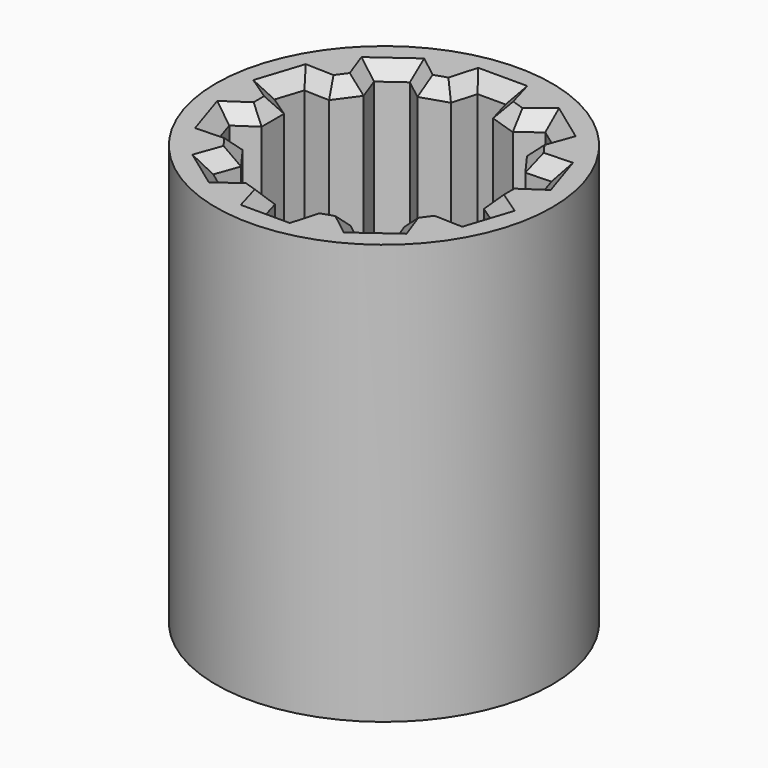
from build123d import *

# Parameters (mm, degrees)
F0_R     = 6
F1_DEPTH = 15
F2_SIZE  = 0.5


# Not quite as in the source:
# - a feature names something its author has since deleted; it is built from what else it names


with BuildPart() as f1:
    # F0 (on Top) → F1 (new body)
    with BuildSketch(Plane.XY):
        Circle(F0_R)
        Polygon((0.5, 4.8), (0.7508449189, 3.9288970345), (1.7019014352, 3.6198800401), (2.4168607138, 4.1771741991), (3.2258777082, 3.5893889469), (2.9167940342, 2.7372089), (3.5045792865, 1.9281919056), (4.410562781, 1.9588098311), (4.7195797754, 1.0077533149), (3.9686269666, 0.5), (3.9686269666, -0.5), (4.7195797754, -1.0077533149), (4.410562781, -1.9588098311), (3.5045792865, -1.9281919056), (2.9167940342, -2.7372089), (3.2258777082, -3.5893889469), (2.4168607138, -4.1771741991), (1.7019014352, -3.6198800401), (0.7508449189, -3.9288970345), (0.5, -4.8), (-0.5, -4.8), (-0.7508449189, -3.9288970345), (-1.7019014352, -3.6198800401), (-2.4168607138, -4.1771741991), (-3.2258777082, -3.5893889469), (-2.9167940342, -2.7372089), (-3.5045792865, -1.9281919056), (-4.410562781, -1.9588098311), (-4.7195797754, -1.0077533149), (-3.9686269666, -0.5), (-3.9686269666, 0.5), (-4.7195797754, 1.0077533149), (-4.410562781, 1.9588098311), (-3.5045792865, 1.9281919056), (-2.9167940342, 2.7372089), (-3.2258777082, 3.5893889469), (-2.4168607138, 4.1771741991), (-1.7019014352, 3.6198800401), (-0.7508449189, 3.9288970345), (-0.5, 4.8), align=None, mode=Mode.SUBTRACT)
    extrude(amount=F1_DEPTH)

    # F2
    f2_edges = [f1.edges().sort_by_distance(p)[0] for p in [
        (-3.071336, -3.163299, 15),
        (-1.226373, -3.774389, 15),
        (-4.565071, -1.483282, 15),
        (-4.565071, 1.483282, 15),
        (-2.821369, -3.883282, 15),
        (-4.344103, 0.753877, 15),
        (2.821369, 3.883282, 15),
        (-0.625422, -4.364449, 15),
        (-3.210687, -2.3327, 15),
        (-3.071336, 3.163299, 15),
        (1.226373, -3.774389, 15),
        (-4.344103, -0.753877, 15),
        (2.059381, 3.898527, 15),
        (3.071336, -3.163299, 15),
        (4.565071, 1.483282, 15),
        (3.957571, 1.943501, 15),
        (3.968627, 0, 15),
        (3.071336, 3.163299, 15),
        (4.344103, 0.753877, 15),
        (2.821369, -3.883282, 15),
        (3.210687, 2.3327, 15),
        (0.625422, 4.364449, 15),
        (-2.059381, 3.898527, 15),
        (0, 4.8, 15),
        (3.957571, -1.943501, 15),
        (2.059381, -3.898527, 15),
        (-3.210687, 2.3327, 15),
        (-0.625422, 4.364449, 15),
        (0.625422, -4.364449, 15),
        (-2.059381, -3.898527, 15),
        (4.344103, -0.753877, 15),
        (3.210687, -2.3327, 15),
        (0, -4.8, 15),
        (-3.968627, 0, 15),
        (-3.957571, -1.943501, 15),
        (4.565071, -1.483282, 15),
        (-2.821369, 3.883282, 15),
        (1.226373, 3.774389, 15),
        (-3.957571, 1.943501, 15),
        (-1.226373, 3.774389, 15),
        (-2.821369, -3.883282, 0),
        (2.821369, -3.883282, 0),
        (0, -4.8, 0),
        (4.344103, -0.753877, 0),
        (1.226373, -3.774389, 0),
        (-4.344103, 0.753877, 0),
        (2.821369, 3.883282, 0),
        (-0.625422, -4.364449, 0),
        (-3.968627, 0, 0),
        (3.957571, -1.943501, 0),
        (-4.565071, -1.483282, 0),
        (-3.071336, -3.163299, 0),
        (-3.071336, 3.163299, 0),
        (-1.226373, -3.774389, 0),
        (-2.059381, 3.898527, 0),
        (-4.565071, 1.483282, 0),
        (0.625422, 4.364449, 0),
        (3.210687, 2.3327, 0),
        (3.957571, 1.943501, 0),
        (1.226373, 3.774389, 0),
        (-3.210687, 2.3327, 0),
        (3.071336, -3.163299, 0),
        (-1.226373, 3.774389, 0),
        (0.625422, -4.364449, 0),
        (-2.821369, 3.883282, 0),
        (-4.344103, -0.753877, 0),
        (-2.059381, -3.898527, 0),
        (4.344103, 0.753877, 0),
        (-0.625422, 4.364449, 0),
        (-3.210687, -2.3327, 0),
        (-3.957571, 1.943501, 0),
        (4.565071, 1.483282, 0),
        (3.968627, 0, 0),
        (2.059381, 3.898527, 0),
        (2.059381, -3.898527, 0),
        (3.210687, -2.3327, 0),
        (0, 4.8, 0),
        (4.565071, -1.483282, 0),
        (3.071336, 3.163299, 0),
        (-3.957571, -1.943501, 0),
    ]]
    chamfer(f2_edges, length=F2_SIZE)


solid = f1.part
